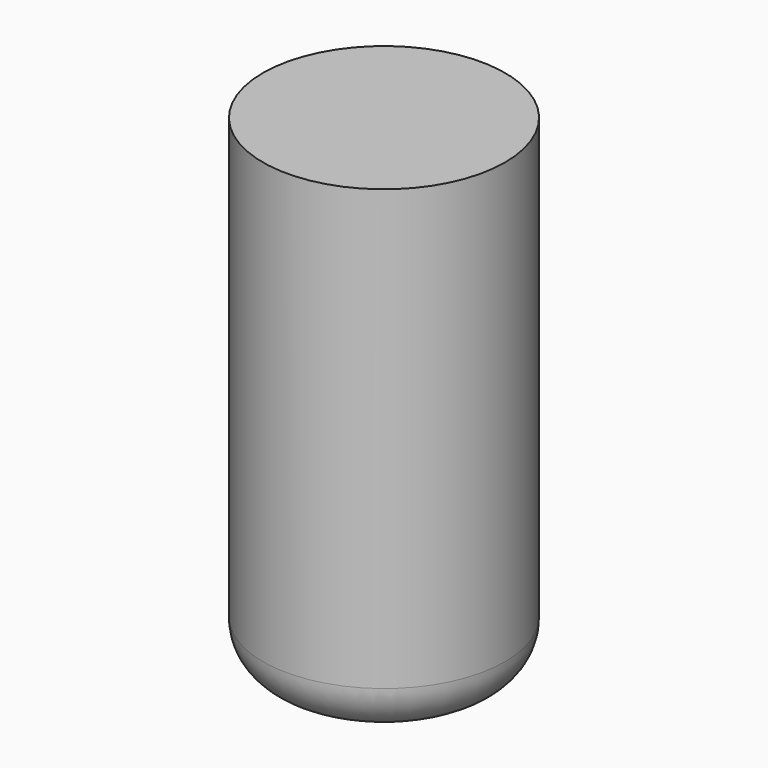
from build123d import *

# Parameters (mm, degrees)
F0_R     = 12.7
F1_DEPTH = 50.8
F3_D     = 19.05
F3_DEPTH = 25.4
F3_TIP   = 5.7231973962


# Not quite as in the source:
# - a fillet or chamfer that OpenCascade refuses, or shapes differently, is made with other operations: its cross-section is extruded or revolved along the edge and cut away or added


with BuildPart() as f1:
    # F0 (on Top) → F1 (new body)
    with BuildSketch(Plane.XY):
        Circle(F0_R)
    extrude(amount=F1_DEPTH)

    # F3
    with Locations(Plane(origin=(0, 0, 0), x_dir=(1, 0, 0), z_dir=(0, 0, -1))):
        with Locations((0, 0)):
            Hole(F3_D / 2, depth=F3_DEPTH)
            with Locations((0, 0, -(F3_DEPTH + F3_TIP / 2))):  # 118° drill point
                Cone(0, F3_D / 2, F3_TIP, mode=Mode.SUBTRACT)

    # F4: fillet of radius 5.08 on 1 edges, made by hand

    # F4_s1 → F4_t2 (revolve, cut)
    with BuildSketch(Plane.XZ):
        with BuildLine():
            ThreePointArc((12.7, 4.7092860393), (11.8321134838, 1.8694797079), (9.525, 0))
            Line((9.525, 0), (12.7, 0))
            Line((12.7, 0), (12.7, 4.7092860393))
        make_face()
    revolve(axis=Axis((0, 0, 0), (0, 0, 1)), mode=Mode.SUBTRACT)


solid = f1.part
